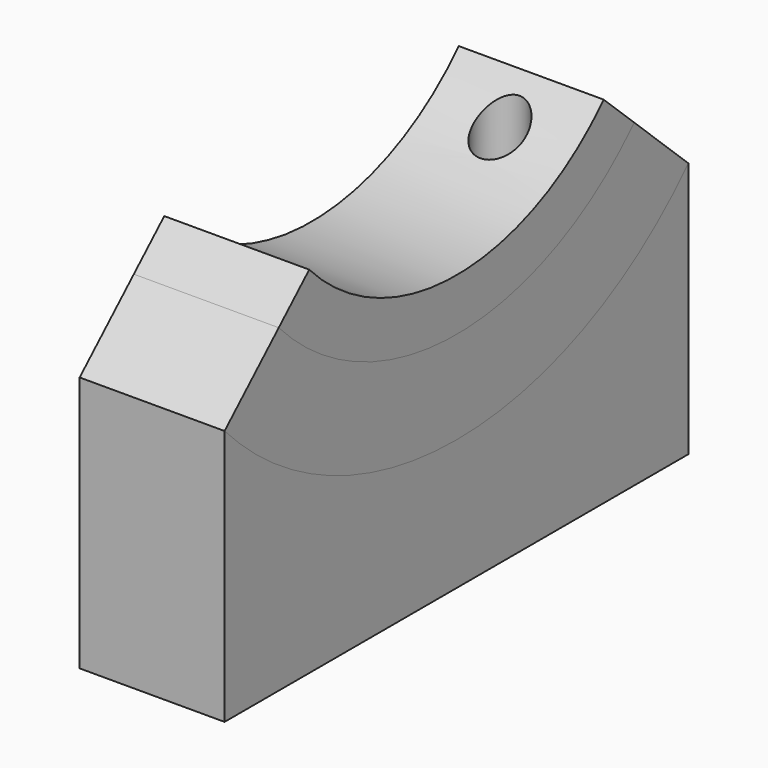
from build123d import *

# Parameters (mm, degrees)
F3_DEPTH  = 25
F4_DEPTH  = 25
F5_DEPTH  = 25
F0_R      = 3
F6_DEPTH  = 61.2676580964
F8_R      = 4.25
F9_DEPTH  = 22.5
F10_DEPTH = 34
F11_DEPTH = 51.5


with BuildPart() as f3:
    # F2 (on plane+point) → F3 (new body)
    with BuildSketch(Plane.YZ.offset(12.5)):
        with BuildLine():
            Line((-50, 0), (50, 0))
            Line((50, 0), (50, 44.1785305656))
            ThreePointArc((50, 44.1785305656), (0, 22.5), (-50, 44.1785305656))
            Line((-50, 44.1785305656), (-50, 0))
        make_face()
    extrude(amount=-F3_DEPTH)


with BuildPart() as f4:
    # F2 (on plane+point) → F4 (new body)
    with BuildSketch(Plane.YZ.offset(12.5)):
        with BuildLine():
            ThreePointArc((-50, 44.1785305656), (0, 22.5), (50, 44.1785305656))
            Line((50, 44.1785305656), (38.3211678832, 55.1149321853))
            ThreePointArc((38.3211678832, 55.1149321853), (0, 38.5), (-38.3211678832, 55.1149321853))
            Line((-38.3211678832, 55.1149321853), (-50, 44.1785305656))
        make_face()
    extrude(amount=-F4_DEPTH)


with BuildPart() as f5:
    # F2 (on plane+point) → F5 (new body)
    with BuildSketch(Plane.YZ.offset(12.5)):
        with BuildLine():
            ThreePointArc((-38.3211678832, 55.1149321853), (0, 38.5), (38.3211678832, 55.1149321853))
            Line((38.3211678832, 55.1149321853), (31.7518248175, 61.2666580964))
            ThreePointArc((31.7518248175, 61.2666580964), (0, 47.5), (-31.7518248175, 61.2666580964))
            Line((-31.7518248175, 61.2666580964), (-38.3211678832, 55.1149321853))
        make_face()
    extrude(amount=-F5_DEPTH)


with BuildPart() as f6_tool:
    # F0 (on Top) → F6 (new body, through all)
    with BuildSketch(Plane.XY):
        with Locations((0, -25)):
            Circle(F0_R)
        with Locations((0, 25)):
            Circle(F0_R)
    extrude(amount=F6_DEPTH)


with BuildPart() as f3_1:
    add(f3.part)

    # F6: cut by f6_tool
    add(f6_tool.part, mode=Mode.SUBTRACT)

    # F8 (on offset) → F11 (cut)
    with BuildSketch(Plane.XY.offset(70)):
        with Locations((0, 25)):
            Circle(F8_R)
        with Locations((0, -25)):
            Circle(F8_R)
    extrude(amount=-F11_DEPTH, mode=Mode.SUBTRACT)


with BuildPart() as f4_1:
    add(f4.part)

    # F6: cut by f6_tool
    add(f6_tool.part, mode=Mode.SUBTRACT)

    # F8 (on offset) → F10 (cut)
    with BuildSketch(Plane.XY.offset(70)):
        with Locations((0, -25)):
            Circle(F8_R)
        with Locations((0, 25)):
            Circle(F8_R)
    extrude(amount=-F10_DEPTH, mode=Mode.SUBTRACT)


with BuildPart() as f5_1:
    add(f5.part)

    # F6: cut by f6_tool
    add(f6_tool.part, mode=Mode.SUBTRACT)

    # F8 (on offset) → F9 (cut)
    with BuildSketch(Plane.XY.offset(70)):
        with Locations((0, -25)):
            Circle(F8_R)
        with Locations((0, 25)):
            Circle(F8_R)
    extrude(amount=-F9_DEPTH, mode=Mode.SUBTRACT)


solid = Compound([f3_1.part, f4_1.part, f5_1.part])
